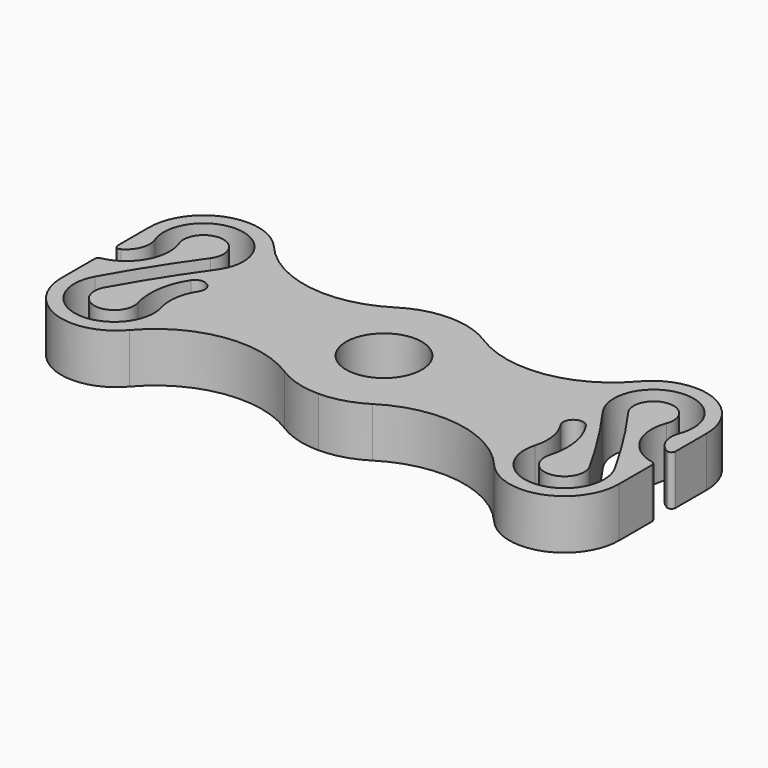
from build123d import *
from build123d import SkipClean  # not in build123d's __all__

# Parameters (mm, degrees)
F1_DEPTH = 25
F3_R     = 2


with BuildPart() as f1:
    # F0 (on Top) → F1 (new body)
    with BuildSketch(Plane.XY):
        with BuildLine():
            ThreePointArc((140, 36), (121, 55), (140, 74))
            Line((140, 74), (140, 96.25))
            ThreePointArc((140, 96.25), (128.4866545127, 94.6106724973), (117.8884190329, 89.8229879123))
            ThreePointArc((117.8884190329, 89.8229879123), (81.203397703, 82.0861941742), (48.4444483171, 100.3207767702))
            ThreePointArc((48.4444483171, 100.3207767702), (18.0058525586, 108.309129477), (0, 82.5))
            Line((0, 82.5), (0, 60))
            ThreePointArc((0, 60), (7.7212902527, 66.0859717551), (8.3025905106, 75.9002198354))
            ThreePointArc((8.3025905106, 75.9002198354), (29.5840689899, 102.832362125), (43.2539034221, 71.3462184874))
            ThreePointArc((43.2539034221, 71.3462184874), (30.1846255305, 51.9598971701), (18.2558114501, 31.8517179024))
            ThreePointArc((18.2558114501, 31.8517179024), (25.8689742306, 17.0641668337), (36.6109152463, 29.7623012378))
            ThreePointArc((36.6109152463, 29.7623012378), (35.6652555644, 44.2047922692), (40.8124091235, 57.7320473369))
            ThreePointArc((40.8124091235, 57.7320473369), (47.7320473369, 59.1875908765), (49.1875908765, 52.2679526631))
            ThreePointArc((49.1875908765, 52.2679526631), (45.5543060113, 42.7193020271), (46.2218304926, 32.5246024755))
            ThreePointArc((46.2218304926, 32.5246024755), (24.7379484611, 7.1283336674), (9.5116229002, 36.7034358047))
            ThreePointArc((9.5116229002, 36.7034358047), (21.7349755999, 57.308113326), (35.1269517111, 77.1731092437))
            ThreePointArc((35.1269517111, 77.1731092437), (28.2920344949, 92.9161810625), (17.6512952553, 79.4501099177))
            ThreePointArc((17.6512952553, 79.4501099177), (16.3752735006, 61.1617226531), (1.6270466845, 50.2721337703))
            ThreePointArc((1.6270466845, 50.2721337703), (0.8248238755, 50.0685027046), (0, 50))
            Line((0, 50), (0, 27.5))
            ThreePointArc((0, 27.5), (18.0058525586, 1.690870523), (48.4444483171, 9.6792232298))
            ThreePointArc((48.4444483171, 9.6792232298), (81.203397703, 27.9138058258), (117.8884190329, 20.1770120877))
            ThreePointArc((117.8884190329, 20.1770120877), (128.4866545127, 15.3893275027), (140, 13.75))
            Line((140, 13.75), (140, 36))
        make_face()
    extrude(amount=F1_DEPTH)

    # F2: F1 across face


with BuildPart() as f1_1:
    add(f1.part, clean=False)
    with SkipClean():  # cleaning this boolean's faces spoils the solid; the shape is the same uncleaned
        add(f1.part.mirror(Plane(origin=(140, 85.125, 12.5), x_dir=(0, 1, 0), z_dir=(1, 0, 0))), clean=False)

    # F3
    f3_edges = [f1_1.edges().sort_by_distance(p)[0] for p in [
        (0, 60, 12.5),
        (0, 50, 12.5),
        (280, 60, 12.5),
        (280, 50, 12.5),
    ]]
    fillet(f3_edges, radius=F3_R)


solid = f1_1.part
